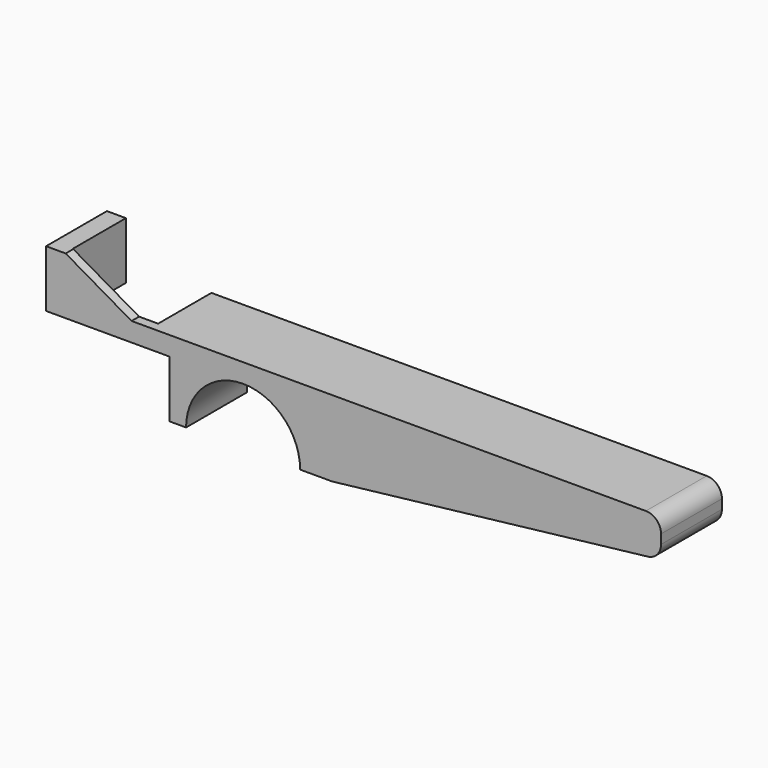
from build123d import *

# Parameters (mm, degrees)
F0_W      = 11.0998
F0_H      = 1.5748
F1_DEPTH  = 12.7
F3_DEPTH  = 9.525
F5_DEPTH  = 6.35
F6_SIZE2  = 10.998513
F6_SIZE   = 6.34999
F7_SIZE   = 3.17499
F8_SIZE   = 2.54
F9_W      = 15.0514596415
F9_H      = 12.7
F10_DEPTH = 25.4
F11_DEPTH = 76.2
F13_DEPTH = 25.4
F15_DEPTH = 25.4
F16_R     = 2.54


# Not quite as in the source:
# - a fillet or chamfer is up to 0.001 mm smaller than in the source, because OpenCascade refuses the exact size


with BuildPart() as f1:
    # F0 (on Top) → F1 (new body)
    with BuildSketch(Plane.XY):
        Polygon((19.0723874551, 12.7), (-4.7528125449, 12.7), (-4.7528125449, 1.5748), (-4.7528125449, 0), (19.0723874551, 0), align=None)
        Polygon((-15.8526125449, 12.7), (-19.0276125449, 12.7), (-19.0276125449, 0), (-15.8526125449, 0), (-15.8526125449, 1.5748), align=None)
        with Locations((-10.3027125449, 0.7874)):
            Rectangle(F0_W, F0_H)
    extrude(amount=F1_DEPTH)

    # F2 (on face) → F3 (cut)
    with BuildSketch(Plane(origin=(0, 0, 0), x_dir=(1, 0, 0), z_dir=(0, 0, -1))):
        Polygon((1.5971874551, -12.7), (1.5971874551, -1.5748), (1.5971874551, 0), (-19.0276125449, 0), (-19.0276125449, -12.7), align=None)
    extrude(amount=-F3_DEPTH, mode=Mode.SUBTRACT)

    # F4 (on face) → F5 (join)
    with BuildSketch(Plane.XY.offset(12.7)):
        Polygon((-15.8526125449, 12.7), (-19.0276125449, 12.7), (-19.0276125449, 0), (-4.7528125449, 0), (-4.7528125449, 1.5748), (-15.8526125449, 1.5748), align=None)
    extrude(amount=F5_DEPTH)

    # F6 (size 6.35 and 10.9985226281 in the source; OpenCascade refuses exactly that, so slightly less here)
    f6_edges = [f1.edges().sort_by_distance(p)[0] for p in [
        (-4.752813, 0.7874, 19.05),
    ]]
    f6_side = f1.faces().sort_by_distance((-4.752813, 0.7874, 15.875))[0]
    chamfer(f6_edges, length=F6_SIZE, length2=F6_SIZE2, reference=f6_side)

    # F7 (size 3.175 in the source; OpenCascade refuses exactly that, so slightly less here)
    f7_edges = [f1.edges().sort_by_distance(p)[0] for p in [
        (-4.752813, 7.1374, 12.7),
    ]]
    chamfer(f7_edges, length=F7_SIZE)

    # F8
    f8_edges = [f1.edges().sort_by_distance(p)[0] for p in [
        (19.072387, 6.35, 12.7),
        (19.072387, 6.35, 0),
        (19.072387, 12.7, 6.35),
    ]]
    chamfer(f8_edges, length=F8_SIZE)

    # F9 (on face) → F10 (cut)
    with BuildSketch(Plane.XY.offset(12.7)):
        with Locations((15.0030172759, 6.35)):
            Rectangle(F9_W, F9_H)
    extrude(amount=-F10_DEPTH, mode=Mode.SUBTRACT)

    # F11 (add): a face of the model
    f11_faces = [f1.faces().sort_by_distance(p)[0] for p in [
        (7.4772874551, 6.35, 6.35),
    ]]
    extrude(f11_faces, amount=F11_DEPTH)

    # F12 (on face) → F13 (cut)
    with BuildSketch(Plane(origin=(0, 12.7, 0), x_dir=(-1, 0, 0), z_dir=(0, 1, 0))):
        with BuildLine():
            Line((-23.4008067042, 0), (-4.3508067042, 0))
            ThreePointArc((-4.3508067042, 0), (-13.8758067042, 9.525), (-23.4008067042, 0))
        make_face()
    extrude(amount=-F13_DEPTH, mode=Mode.SUBTRACT)

    # F14 (on face) → F15 (cut)
    with BuildSketch(Plane(origin=(0, 12.7, 0), x_dir=(-1, 0, 0), z_dir=(0, 1, 0))):
        Polygon((-83.6772874551, 0), (-28.7684481591, 0), (-83.6772874551, 6.35), align=None)
    extrude(amount=-F15_DEPTH, mode=Mode.SUBTRACT)

    # F16
    f16_edges = [f1.edges().sort_by_distance(p)[0] for p in [
        (83.677287, 6.35, 12.7),
        (83.677287, 6.35, 6.35),
    ]]
    fillet(f16_edges, radius=F16_R)


solid = f1.part
